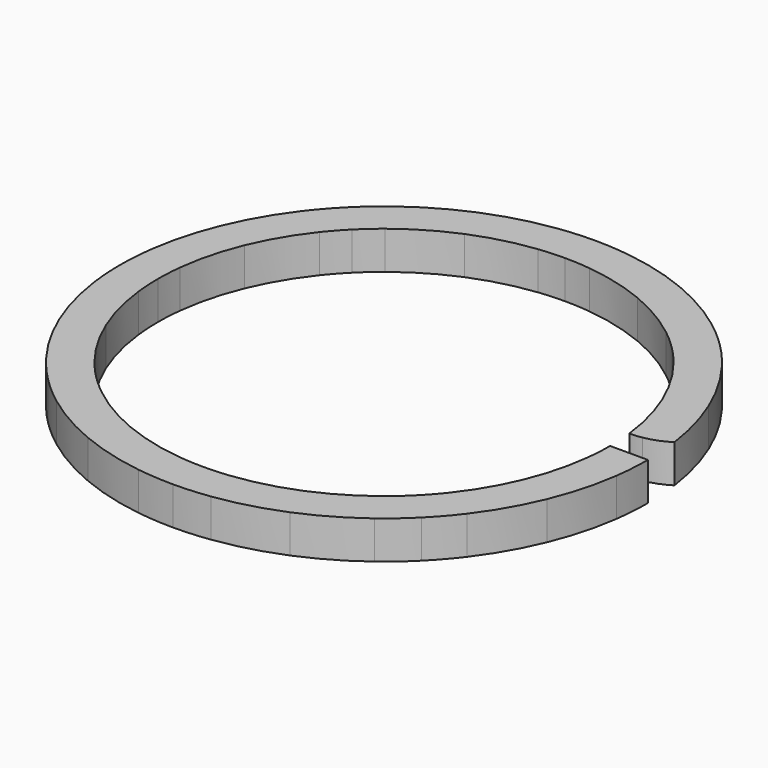
from build123d import *

# Parameters (mm, degrees)
F2_DEPTH = 2


with BuildPart() as f2:
    # F1 (on face) → F2 (new body)
    with BuildSketch(Plane.XY):
        with BuildLine():
            ThreePointArc((18.3001549066, -2.0420113713), (17.9462510765, -0.3112895728), (17.3754329945, 1.3604797241))
            Line((17.3754329945, 1.3604797241), (15.5377167825, 0.5992727453))
            ThreePointArc((15.5377167825, 0.5992727453), (16.0627067105, -0.968422059), (16.3652392751, -2.593769859))
            ThreePointArc((16.3652392751, -2.593769859), (16.6935081093, -2.5817022248), (17.0192561264, -2.5393432276))
            ThreePointArc((17.0192561264, -2.5393432276), (17.6839972454, -2.3532416527), (18.3001549066, -2.0420113713))
        make_face()
        with BuildLine():
            Line((15.5377167825, 0.5992727453), (17.3754329945, 1.3604797241))
            ThreePointArc((17.3754329945, 1.3604797241), (16.5969429247, 2.9462284671), (15.6233856027, 4.4202813853))
            ThreePointArc((15.6233856027, 4.4202813853), (14.6734726061, 4.0584412817), (13.8650414705, 3.4422415894))
            ThreePointArc((13.8650414705, 3.4422415894), (14.8004130937, 2.0790243103), (15.5377167825, 0.5992727453))
        make_face()
        with BuildLine():
            ThreePointArc((13.8650414705, 3.4422415894), (14.6734726061, 4.0584412817), (15.6233856027, 4.4202813853))
            ThreePointArc((15.6233856027, 4.4202813853), (15.0196144043, 5.16406253), (14.3659866612, 5.8644344489))
            Line((14.3659866612, 5.8644344489), (12.9594595658, 4.4579073535))
            ThreePointArc((12.9594595658, 4.4579073535), (13.4267875285, 3.9630358747), (13.8650414705, 3.4422415894))
        make_face()
        with BuildLine():
            ThreePointArc((18.3001549066, -5.8625828565), (18.399156889, -4.9097194566), (18.4322100127, -3.9522971139))
            Line((18.4322100127, -3.9522971139), (16.4430803185, -3.9522971139))
            ThreePointArc((16.4430803185, -3.9522971139), (16.4236041115, -4.6326748639), (16.3652392751, -5.3108243689))
            ThreePointArc((16.3652392751, -5.3108243689), (17.3726053942, -5.446752526), (18.3001549066, -5.8625828565))
        make_face()
        with BuildLine():
            Line((12.9594595658, 4.4579073535), (14.3659866612, 5.8644344489))
            ThreePointArc((14.3659866612, 5.8644344489), (13.6656147423, 6.518062192), (12.9218335976, 7.1218333904))
            ThreePointArc((12.9218335976, 7.1218333904), (12.559993494, 6.1719203938), (11.9437938017, 5.3634892582))
            ThreePointArc((11.9437938017, 5.3634892582), (12.464588087, 4.9252353162), (12.9594595658, 4.4579073535))
        make_face()
        with BuildLine():
            ThreePointArc((17.3754329945, -9.2650739519), (17.9462510765, -7.593304655), (18.3001549066, -5.8625828565))
            ThreePointArc((18.3001549066, -5.8625828565), (17.3726053942, -5.446752526), (16.3652392751, -5.3108243689))
            ThreePointArc((16.3652392751, -5.3108243689), (16.0627067105, -6.9361721689), (15.5377167825, -8.5038669731))
            Line((15.5377167825, -8.5038669731), (17.3754329945, -9.2650739519))
        make_face()
        with BuildLine():
            ThreePointArc((11.9437938017, 5.3634892582), (12.559993494, 6.1719203938), (12.9218335976, 7.1218333904))
            ThreePointArc((12.9218335976, 7.1218333904), (11.4477806794, 8.0953907124), (9.8620319364, 8.8738807822))
            Line((9.8620319364, 8.8738807822), (9.1008249576, 7.0361645702))
            ThreePointArc((9.1008249576, 7.0361645702), (10.5805765226, 6.2988608814), (11.9437938017, 5.3634892582))
        make_face()
        with BuildLine():
            ThreePointArc((15.6233856027, -12.3248756131), (16.5969429247, -10.8508226949), (17.3754329945, -9.2650739519))
            Line((17.3754329945, -9.2650739519), (15.5377167825, -8.5038669731))
            ThreePointArc((15.5377167825, -8.5038669731), (14.8004130937, -9.9836185381), (13.8650414705, -11.3468358173))
            ThreePointArc((13.8650414705, -11.3468358173), (14.6734726061, -11.9630355095), (15.6233856027, -12.3248756131))
        make_face()
        with BuildLine():
            Line((9.1008249576, 7.0361645702), (9.8620319364, 8.8738807822))
            ThreePointArc((9.8620319364, 8.8738807822), (8.1902626395, 9.4446988642), (6.459540841, 9.7986026942))
            ThreePointArc((6.459540841, 9.7986026942), (6.0437105105, 8.8710531819), (5.9077823533, 7.8636870628))
            ThreePointArc((5.9077823533, 7.8636870628), (7.5331301533, 7.5611544982), (9.1008249576, 7.0361645702))
        make_face()
        with BuildLine():
            ThreePointArc((14.3659866612, -13.7690286767), (15.0196144043, -13.0686567579), (15.6233856027, -12.3248756131))
            ThreePointArc((15.6233856027, -12.3248756131), (14.6734726061, -11.9630355095), (13.8650414705, -11.3468358173))
            ThreePointArc((13.8650414705, -11.3468358173), (13.4267875285, -11.8676301025), (12.9594595658, -12.3625015813))
            Line((12.9594595658, -12.3625015813), (14.3659866612, -13.7690286767))
        make_face()
        with BuildLine():
            ThreePointArc((5.9077823533, 7.8636870628), (6.0437105105, 8.8710531819), (6.459540841, 9.7986026942))
            ThreePointArc((6.459540841, 9.7986026942), (5.5066774411, 9.8976046767), (4.5492550984, 9.9306578004))
            Line((4.5492550984, 9.9306578004), (4.5492550984, 7.9415281062))
            ThreePointArc((4.5492550984, 7.9415281062), (5.2296328483, 7.9220518992), (5.9077823533, 7.8636870628))
        make_face()
        with BuildLine():
            ThreePointArc((12.9218335976, -15.0264276183), (13.6656147423, -14.4226564199), (14.3659866612, -13.7690286767))
            Line((14.3659866612, -13.7690286767), (12.9594595658, -12.3625015813))
            ThreePointArc((12.9594595658, -12.3625015813), (12.464588087, -12.829829544), (11.9437938017, -13.2680834861))
            ThreePointArc((11.9437938017, -13.2680834861), (12.559993494, -14.0765146217), (12.9218335976, -15.0264276183))
        make_face()
        with BuildLine():
            Line((4.5492550984, 7.9415281062), (4.5492550984, 9.9306578004))
            ThreePointArc((4.5492550984, 9.9306578004), (3.5918327557, 9.8976046767), (2.6389693558, 9.7986026942))
            ThreePointArc((2.6389693558, 9.7986026942), (3.0547996863, 8.8710531819), (3.1907278434, 7.8636870628))
            ThreePointArc((3.1907278434, 7.8636870628), (3.8688773484, 7.9220518992), (4.5492550984, 7.9415281062))
        make_face()
        with BuildLine():
            ThreePointArc((9.8620319364, -16.77847501), (11.4477806794, -15.9999849403), (12.9218335976, -15.0264276183))
            ThreePointArc((12.9218335976, -15.0264276183), (12.559993494, -14.0765146217), (11.9437938017, -13.2680834861))
            ThreePointArc((11.9437938017, -13.2680834861), (10.5805765226, -14.2034551093), (9.1008249576, -14.9407587981))
            Line((9.1008249576, -14.9407587981), (9.8620319364, -16.77847501))
        make_face()
        with BuildLine():
            ThreePointArc((3.1907278434, 7.8636870628), (3.0547996863, 8.8710531819), (2.6389693558, 9.7986026942))
            ThreePointArc((2.6389693558, 9.7986026942), (0.9082475573, 9.4446988642), (-0.7635217396, 8.8738807822))
            Line((-0.7635217396, 8.8738807822), (-0.0023147608, 7.0361645702))
            ThreePointArc((-0.0023147608, 7.0361645702), (1.5653800434, 7.5611544982), (3.1907278434, 7.8636870628))
        make_face()
        with BuildLine():
            ThreePointArc((6.459540841, -17.7031969221), (8.1902626395, -17.3492930921), (9.8620319364, -16.77847501))
            Line((9.8620319364, -16.77847501), (9.1008249576, -14.9407587981))
            ThreePointArc((9.1008249576, -14.9407587981), (7.5331301533, -15.465748726), (5.9077823533, -15.7682812907))
            ThreePointArc((5.9077823533, -15.7682812907), (6.0437105105, -16.7756474097), (6.459540841, -17.7031969221))
        make_face()
        with BuildLine():
            Line((-0.0023147608, 7.0361645702), (-0.7635217396, 8.8738807822))
            ThreePointArc((-0.7635217396, 8.8738807822), (-2.3492704826, 8.0953907124), (-3.8233234008, 7.1218333904))
            ThreePointArc((-3.8233234008, 7.1218333904), (-3.4614832972, 6.1719203938), (-2.845283605, 5.3634892582))
            ThreePointArc((-2.845283605, 5.3634892582), (-1.4820663258, 6.2988608814), (-0.0023147608, 7.0361645702))
        make_face()
        with BuildLine():
            ThreePointArc((4.5492550984, -17.8352520282), (5.5066774411, -17.8021989046), (6.459540841, -17.7031969221))
            ThreePointArc((6.459540841, -17.7031969221), (6.0437105105, -16.7756474097), (5.9077823533, -15.7682812907))
            ThreePointArc((5.9077823533, -15.7682812907), (5.2296328483, -15.826646127), (4.5492550984, -15.8461223341))
            Line((4.5492550984, -15.8461223341), (4.5492550984, -17.8352520282))
        make_face()
        with BuildLine():
            ThreePointArc((-2.845283605, 5.3634892582), (-3.4614832972, 6.1719203938), (-3.8233234008, 7.1218333904))
            ThreePointArc((-3.8233234008, 7.1218333904), (-4.5671045455, 6.518062192), (-5.2674764644, 5.8644344489))
            Line((-5.2674764644, 5.8644344489), (-3.860949369, 4.4579073535))
            ThreePointArc((-3.860949369, 4.4579073535), (-3.3660778902, 4.9252353162), (-2.845283605, 5.3634892582))
        make_face()
        with BuildLine():
            ThreePointArc((2.6389693558, -17.7031969221), (3.5918327557, -17.8021989046), (4.5492550984, -17.8352520282))
            Line((4.5492550984, -17.8352520282), (4.5492550984, -15.8461223341))
            ThreePointArc((4.5492550984, -15.8461223341), (3.8688773484, -15.826646127), (3.1907278434, -15.7682812907))
            ThreePointArc((3.1907278434, -15.7682812907), (3.0547996863, -16.7756474097), (2.6389693558, -17.7031969221))
        make_face()
        with BuildLine():
            Line((-3.860949369, 4.4579073535), (-5.2674764644, 5.8644344489))
            ThreePointArc((-5.2674764644, 5.8644344489), (-5.9211042076, 5.16406253), (-6.524875406, 4.4202813853))
            ThreePointArc((-6.524875406, 4.4202813853), (-5.5749624094, 4.0584412817), (-4.7665312738, 3.4422415894))
            ThreePointArc((-4.7665312738, 3.4422415894), (-4.3282773317, 3.9630358747), (-3.860949369, 4.4579073535))
        make_face()
        with BuildLine():
            ThreePointArc((-0.7635217396, -16.77847501), (0.9082475573, -17.3492930921), (2.6389693558, -17.7031969221))
            ThreePointArc((2.6389693558, -17.7031969221), (3.0547996863, -16.7756474097), (3.1907278434, -15.7682812907))
            ThreePointArc((3.1907278434, -15.7682812907), (1.5653800434, -15.465748726), (-0.0023147608, -14.9407587981))
            Line((-0.0023147608, -14.9407587981), (-0.7635217396, -16.77847501))
        make_face()
        with BuildLine():
            ThreePointArc((-4.7665312738, 3.4422415894), (-5.5749624094, 4.0584412817), (-6.524875406, 4.4202813853))
            ThreePointArc((-6.524875406, 4.4202813853), (-7.498432728, 2.9462284671), (-8.2769227977, 1.3604797241))
            Line((-8.2769227977, 1.3604797241), (-6.4392065858, 0.5992727453))
            ThreePointArc((-6.4392065858, 0.5992727453), (-5.701902897, 2.0790243103), (-4.7665312738, 3.4422415894))
        make_face()
        with BuildLine():
            ThreePointArc((-3.8233234008, -15.0264276183), (-2.3492704826, -15.9999849403), (-0.7635217396, -16.77847501))
            Line((-0.7635217396, -16.77847501), (-0.0023147608, -14.9407587981))
            ThreePointArc((-0.0023147608, -14.9407587981), (-1.4820663258, -14.2034551093), (-2.845283605, -13.2680834861))
            ThreePointArc((-2.845283605, -13.2680834861), (-3.4614832972, -14.0765146217), (-3.8233234008, -15.0264276183))
        make_face()
        with BuildLine():
            Line((-6.4392065858, 0.5992727453), (-8.2769227977, 1.3604797241))
            ThreePointArc((-8.2769227977, 1.3604797241), (-8.8477408798, -0.3112895728), (-9.2016447098, -2.0420113713))
            ThreePointArc((-9.2016447098, -2.0420113713), (-8.2740951974, -2.4578417018), (-7.2667290784, -2.593769859))
            ThreePointArc((-7.2667290784, -2.593769859), (-6.9641965137, -0.968422059), (-6.4392065858, 0.5992727453))
        make_face()
        with BuildLine():
            ThreePointArc((-5.2674764644, -13.7690286767), (-4.5671045455, -14.4226564199), (-3.8233234008, -15.0264276183))
            ThreePointArc((-3.8233234008, -15.0264276183), (-3.4614832972, -14.0765146217), (-2.845283605, -13.2680834861))
            ThreePointArc((-2.845283605, -13.2680834861), (-3.3660778902, -12.829829544), (-3.860949369, -12.3625015813))
            Line((-3.860949369, -12.3625015813), (-5.2674764644, -13.7690286767))
        make_face()
        with BuildLine():
            ThreePointArc((-7.2667290784, -2.593769859), (-8.2740951974, -2.4578417018), (-9.2016447098, -2.0420113713))
            ThreePointArc((-9.2016447098, -2.0420113713), (-9.3006466923, -2.9948747712), (-9.3336998159, -3.9522971139))
            Line((-9.3336998159, -3.9522971139), (-7.3445701218, -3.9522971139))
            ThreePointArc((-7.3445701218, -3.9522971139), (-7.3250939147, -3.271919364), (-7.2667290784, -2.593769859))
        make_face()
        with BuildLine():
            ThreePointArc((-6.524875406, -12.3248756131), (-5.9211042076, -13.0686567579), (-5.2674764644, -13.7690286767))
            Line((-5.2674764644, -13.7690286767), (-3.860949369, -12.3625015813))
            ThreePointArc((-3.860949369, -12.3625015813), (-4.3282773317, -11.8676301025), (-4.7665312738, -11.3468358173))
            ThreePointArc((-4.7665312738, -11.3468358173), (-5.5749624094, -11.9630355095), (-6.524875406, -12.3248756131))
        make_face()
        with BuildLine():
            Line((-7.3445701218, -3.9522971139), (-9.3336998159, -3.9522971139))
            ThreePointArc((-9.3336998159, -3.9522971139), (-9.3006466923, -4.9097194566), (-9.2016447098, -5.8625828565))
            ThreePointArc((-9.2016447098, -5.8625828565), (-8.2740951974, -5.446752526), (-7.2667290784, -5.3108243689))
            ThreePointArc((-7.2667290784, -5.3108243689), (-7.3250939147, -4.6326748639), (-7.3445701218, -3.9522971139))
        make_face()
        with BuildLine():
            ThreePointArc((-8.2769227977, -9.2650739519), (-7.498432728, -10.8508226949), (-6.524875406, -12.3248756131))
            ThreePointArc((-6.524875406, -12.3248756131), (-5.5749624094, -11.9630355095), (-4.7665312738, -11.3468358173))
            ThreePointArc((-4.7665312738, -11.3468358173), (-5.701902897, -9.9836185381), (-6.4392065858, -8.5038669731))
            Line((-6.4392065858, -8.5038669731), (-8.2769227977, -9.2650739519))
        make_face()
        with BuildLine():
            ThreePointArc((-7.2667290784, -5.3108243689), (-8.2740951974, -5.446752526), (-9.2016447098, -5.8625828565))
            ThreePointArc((-9.2016447098, -5.8625828565), (-8.8477408798, -7.593304655), (-8.2769227977, -9.2650739519))
            Line((-8.2769227977, -9.2650739519), (-6.4392065858, -8.5038669731))
            ThreePointArc((-6.4392065858, -8.5038669731), (-6.9641965137, -6.9361721689), (-7.2667290784, -5.3108243689))
        make_face()
    extrude(amount=F2_DEPTH)


solid = f2.part
